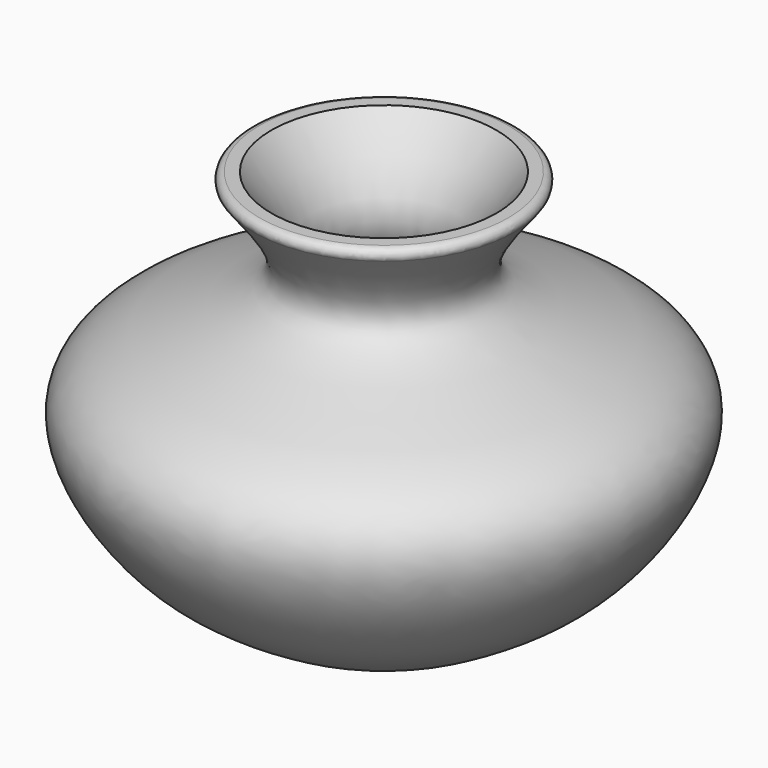
from build123d import *

# Parameters (mm, degrees)
F2_R = 1
F3_T = 3


# Not quite as in the source:
# - a shell that OpenCascade refuses in one call is made with other operations: the cavity is built on its own and cut out


with BuildPart() as f1:
    # F0 (on Front) → F1 (revolve)
    with BuildSketch(Plane.XZ):
        with BuildLine():
            Line((0, 53.6803081632), (0, 0))
            Line((0, 0), (19.687499851, 0))
            add(Edge.make_bspline(
                [(20.2540475875, 53.6803081632), (18.6384112126, 51.7463255353), (15.4691397035, 47.9525782934), (9.9343595071, 38.0617206442), (33.3312284292, 33.1846739682), (41.201877378, 22.7552228995), (31.298748703, 6.7755111019), (23.4415391534, 2.19059425), (19.687499851, 0)],
                knots=[0, 0, 0, 0, 0.1331516095, 0.2611934274, 0.4741420117, 0.632665789, 0.824494045, 1, 1, 1, 1], degree=3))
            Line((20.2540475875, 53.6803081632), (0, 53.6803081632))
        make_face()
    revolve(axis=Axis((0, 0, 29.6728890389), (0, 0, 1)))

    # F2
    f2_edges = [f1.edges().sort_by_distance(p)[0] for p in [
        (-20.254048, 0, 53.680308),
    ]]
    fillet(f2_edges, radius=F2_R)

    # F3: shell of thickness 3, made by hand


with BuildPart() as f3_core1:
    # F3_t2: copy of F1
    add(f1.part)

    # the walls: a layer under each face that stays
    f3_faces = [f3_core1.faces().sort_by_distance(p)[0] for p in [
        (-35.0774831473, 0, 29.4661465552),
        (-19.0281361236, 0, 53.1080918413),
        (0, 0, 0),
    ]]
    thicken(f3_faces, amount=-F3_T, mode=Mode.SUBTRACT)


with BuildPart() as f1_1:
    add(f1.part)

    # what is left inside the walls is the cavity
    f3_cavity = [f3_core1.part.solids().sort_by_distance(p)[0] for p in [
        (-19.363052, 0, 33.363934),
    ]]
    add(f3_cavity, mode=Mode.SUBTRACT)


solid = f1_1.part
